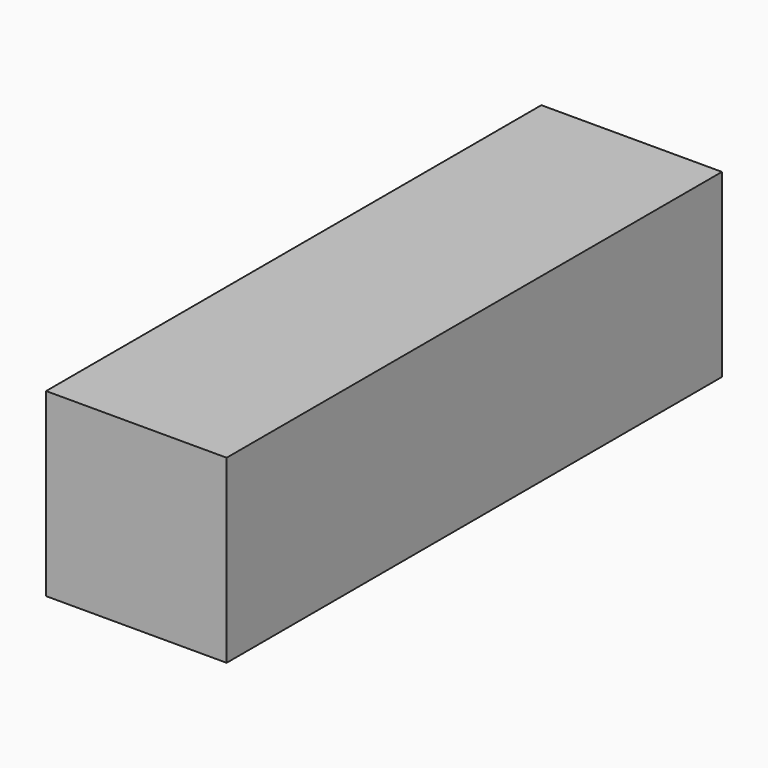
from build123d import *

# Parameters (mm, degrees)
F0_W     = 88.9
F0_H     = 88.9
F2_DEPTH = 304.8


# Not quite as in the source:
# - a variable given as a bare number and used for a length is read in inches; the dataset says mm whatever the document's units were


with BuildPart() as f2:
    # F0 (on Front) → F2 (new body)
    with BuildSketch(Plane.XZ):
        with Locations((44.45, 44.45)):
            Rectangle(F0_W, F0_H)
    extrude(amount=-F2_DEPTH)


solid = f2.part
